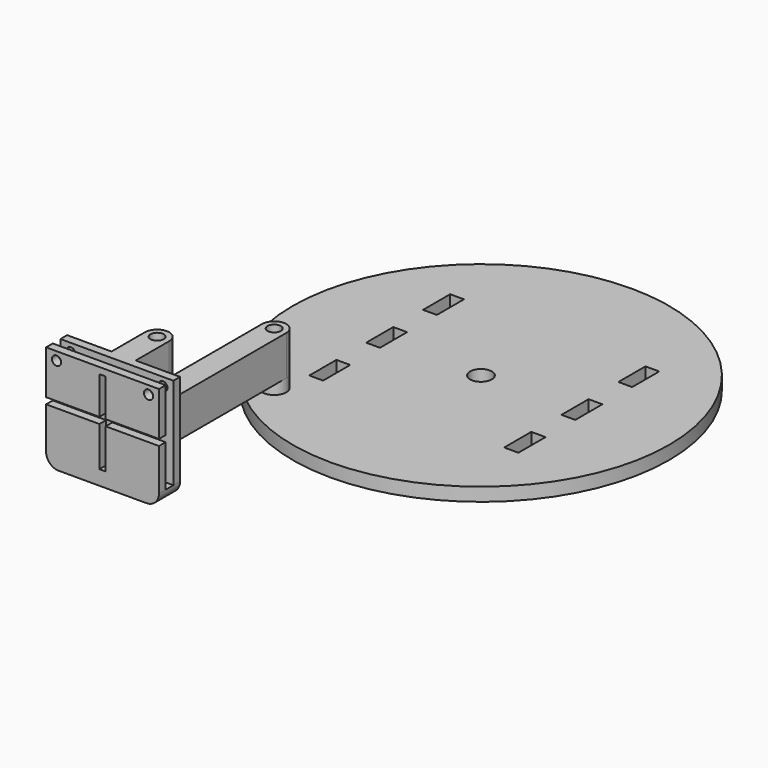
from build123d import *

# Parameters (mm, degrees)
F0_R      = 2.6
F1_DEPTH  = 3.2
F2_R      = 45
F2_R_2    = 35.3553390593
F3_DEPTH  = 3.2
F4_R      = 1.6
F5_DEPTH  = 3.2
F4_R_2    = 2.9
F6_DEPTH  = 2.5
F7_DEPTH  = 12
F9_DEPTH  = 3
F10_R     = 1.6
F11_DEPTH = 9.5
F12_R     = 12.5
F12_R_2   = 2.6
F13_DEPTH = 3.2
F14_R     = 1.6
F15_DEPTH = 12.5
F16_W     = 27
F16_H     = 2
F16_W_2   = 12.75
F16_W_3   = 1.5
F17_DEPTH = 25
F18_R     = 3
F19_DEPTH = 22
F20_DEPTH = 12
F21_DEPTH = 21.5
F22_R     = 1.1
F23_DEPTH = 2
F24_R     = 1.1
F25_DEPTH = 2


# Not quite as in the source:
# - a feature names something its author has since deleted; it is built from what else it names


with BuildPart() as f1:
    # F0 (on Top) → F1 (new body)
    with BuildSketch(Plane.XY):
        with BuildLine():
            ThreePointArc((25, -25), (32.6640741219, -13.5299025037), (35.3553390593, 0))
            ThreePointArc((35.3553390593, 0), (32.6640741219, 13.5299025037), (25, 25))
            Line((25, 25), (25, 22.05))
            Line((25, 22.05), (25, 13.95))
            Line((25, 13.95), (25, 5.05))
            Line((25, 5.05), (25, -3.05))
            Line((25, -3.05), (25, -11.95))
            Line((25, -11.95), (25, -20.05))
            Line((25, -20.05), (25, -25))
        make_face()
        with BuildLine():
            Line((-25, 25), (25, 25))
            ThreePointArc((25, 25), (0, 35.3553390593), (-25, 25))
        make_face()
        Polygon((25, 22.05), (25, 25), (-25, 25), (-25, 22.05), (-21.7, 22.05), (-21.7, 13.95), (-25, 13.95), (-25, 5.05), (-21.7, 5.05), (-21.7, -3.05), (-25, -3.05), (-25, -11.95), (-21.7, -11.95), (-21.7, -20.05), (-25, -20.05), (-25, -25), (25, -25), (25, -20.05), (21.6, -20.05), (21.6, -11.95), (25, -11.95), (25, -3.05), (21.7, -3.05), (21.7, 5.05), (25, 5.05), (25, 13.95), (21.7, 13.95), (21.7, 22.05), align=None)
        Circle(F0_R, mode=Mode.SUBTRACT)
        with BuildLine():
            ThreePointArc((-25, -25), (0, -35.3553390593), (25, -25))
            Line((25, -25), (-25, -25))
        make_face()
        with BuildLine():
            Line((-25, 22.05), (-25, 25))
            ThreePointArc((-25, 25), (-35.3553390593, 0), (-25, -25))
            Line((-25, -25), (-25, -20.05))
            Line((-25, -20.05), (-25, -11.95))
            Line((-25, -11.95), (-25, -3.05))
            Line((-25, -3.05), (-25, 5.05))
            Line((-25, 5.05), (-25, 13.95))
            Line((-25, 13.95), (-25, 22.05))
        make_face()
    extrude(amount=F1_DEPTH)

    # F2 (on Top) → F3 (join, through all)
    with BuildSketch(Plane.XY):
        Circle(F2_R)
        Circle(F2_R_2, mode=Mode.SUBTRACT)
    extrude(amount=F3_DEPTH)

    # F4 (on face) → F5 (cut, through all)
    with BuildSketch(Plane.XY.offset(3.2)):
        with Locations((-27, -28.05)):
            Circle(F4_R)
    extrude(amount=-F5_DEPTH, mode=Mode.SUBTRACT)


with BuildPart() as f6:
    # F4 (on face) → F6 (new body)
    with BuildSketch(Plane.XY.offset(3.2)):
        with Locations((-27, -28.05)):
            Circle(F4_R_2)
        with Locations((-27, -28.05)):
            Circle(F4_R, mode=Mode.SUBTRACT)
    extrude(amount=F6_DEPTH)


with BuildPart() as f7:
    # F4 (on face) → F7 (new body)
    with BuildSketch(Plane.XY.offset(3.2)):
        with Locations((-27, -28.05)):
            Circle(F4_R_2)
        with Locations((-27, -28.05)):
            Circle(F4_R, mode=Mode.SUBTRACT)
    extrude(amount=F7_DEPTH)


with BuildPart() as f9:
    # F4 (on face) → F9 (new body)
    with BuildSketch(Plane.XY.offset(3.2)):
        with Locations((-27, -28.05)):
            Circle(F4_R_2)
        with Locations((-27, -28.05)):
            Circle(F4_R, mode=Mode.SUBTRACT)
    extrude(amount=F9_DEPTH)


with BuildPart() as f11:
    # F10 (on face) → F11 (new body)
    with BuildSketch(Plane.XY.offset(6.2)):
        with BuildLine():
            ThreePointArc((-29.9, -28.05), (-27, -30.95), (-24.1, -28.05))
            ThreePointArc((-24.1, -28.05), (-27, -25.15), (-29.9, -28.05))
        make_face()
        with Locations((-27, -28.05)):
            Circle(F10_R, mode=Mode.SUBTRACT)
        with BuildLine():
            Line((-24.1, -63.05), (-24.1, -28.05))
            ThreePointArc((-24.1, -28.05), (-27, -30.95), (-29.9, -28.05))
            Line((-29.9, -28.05), (-29.9, -63.05))
            ThreePointArc((-29.9, -63.05), (-27, -60.15), (-24.1, -63.05))
        make_face()
        with BuildLine():
            ThreePointArc((-29.9, -63.05), (-27, -65.95), (-24.1, -63.05))
            ThreePointArc((-24.1, -63.05), (-27, -60.15), (-29.9, -63.05))
        make_face()
        with Locations((-27, -63.05)):
            Circle(F10_R, mode=Mode.SUBTRACT)
    extrude(amount=F11_DEPTH)


with BuildPart() as f13:
    # F12 (on face) → F13 (new body)
    with BuildSketch(Plane(origin=(0, 0, 0), x_dir=(1, 0, 0), z_dir=(0, 0, -1))):
        Circle(F12_R)
        Circle(F12_R_2, mode=Mode.SUBTRACT)
    extrude(amount=F13_DEPTH)


with BuildPart() as f15:
    # F14 (on face) → F15 (new body)
    with BuildSketch(Plane.XY.offset(15.7)):
        with BuildLine():
            ThreePointArc((-29.9, -63.05), (-27, -65.95), (-24.1, -63.05))
            ThreePointArc((-24.1, -63.05), (-27, -60.15), (-29.9, -63.05))
        make_face()
        with Locations((-27, -63.05)):
            Circle(F14_R, mode=Mode.SUBTRACT)
        with BuildLine():
            Line((-24.1, -73.05), (-24.1, -63.05))
            ThreePointArc((-24.1, -63.05), (-27, -65.95), (-29.9, -63.05))
            Line((-29.9, -63.05), (-29.9, -73.05))
            Line((-29.9, -73.05), (-24.1, -73.05))
        make_face()
    extrude(amount=F15_DEPTH)

    # F16 (on face) → F17 (join)
    with BuildSketch(Plane.XY.offset(28.2)):
        with Locations((-27, -74.05)):
            Rectangle(F16_W, F16_H)
        Polygon((-13.5, -75.05), (-40.5, -75.05), (-40.5, -77.35), (-27.75, -77.35), (-26.25, -77.35), (-13.5, -77.35), align=None)
        with Locations((-34.125, -78.35)):
            Rectangle(F16_W_2, F16_H)
        with Locations((-19.875, -78.35)):
            Rectangle(F16_W_2, F16_H)
        with Locations((-27, -78.35)):
            Rectangle(F16_W_3, F16_H)
    extrude(amount=-F17_DEPTH)

    # F18
    f18_edges = [f15.edges().sort_by_distance(p)[0] for p in [
        (-40.5, -76.2, 3.2),
        (-13.5, -76.2, 3.2),
    ]]
    fillet(f18_edges, radius=F18_R)

    # F16 (on face) → F19 (cut)
    with BuildSketch(Plane.XY.offset(28.2)):
        Polygon((-13.5, -75.05), (-40.5, -75.05), (-40.5, -77.35), (-27.75, -77.35), (-26.25, -77.35), (-13.5, -77.35), align=None)
    extrude(amount=-F19_DEPTH, mode=Mode.SUBTRACT)

    # F16 (on face) → F20 (cut)
    with BuildSketch(Plane.XY.offset(28.2)):
        with Locations((-34.125, -78.35)):
            Rectangle(F16_W_2, F16_H)
        with Locations((-27, -78.35)):
            Rectangle(F16_W_3, F16_H)
        with Locations((-19.875, -78.35)):
            Rectangle(F16_W_2, F16_H)
    extrude(amount=-F20_DEPTH, mode=Mode.SUBTRACT)

    # F16 (on face) → F21 (cut)
    with BuildSketch(Plane.XY.offset(28.2)):
        with Locations((-27, -78.35)):
            Rectangle(F16_W_3, F16_H)
    extrude(amount=-F21_DEPTH, mode=Mode.SUBTRACT)

    # F24 (on face) → F25 (cut, through all)
    with BuildSketch(Plane.XZ.offset(75.05)):
        with Locations((-38, 26.2)):
            Circle(F24_R)
        with Locations((-16, 26.2)):
            Circle(F24_R)
    extrude(amount=-F25_DEPTH, mode=Mode.SUBTRACT)


with BuildPart() as f23:
    # F22 (on face) → F23 (new body, through all)
    with BuildSketch(Plane.XZ.offset(79.35)):
        Polygon((-40.5, 17.7), (-27.75, 17.7), (-27.75, 26.7), (-26.25, 26.7), (-26.25, 17.7), (-13.5, 17.7), (-13.5, 28.2), (-40.5, 28.2), align=None)
        with Locations((-38, 26.2)):
            Circle(F22_R, mode=Mode.SUBTRACT)
        with Locations((-16, 26.2)):
            Circle(F22_R, mode=Mode.SUBTRACT)
    extrude(amount=-F23_DEPTH)


solid = Compound([f1.part, f9.part, f11.part, f13.part, f15.part, f23.part])
